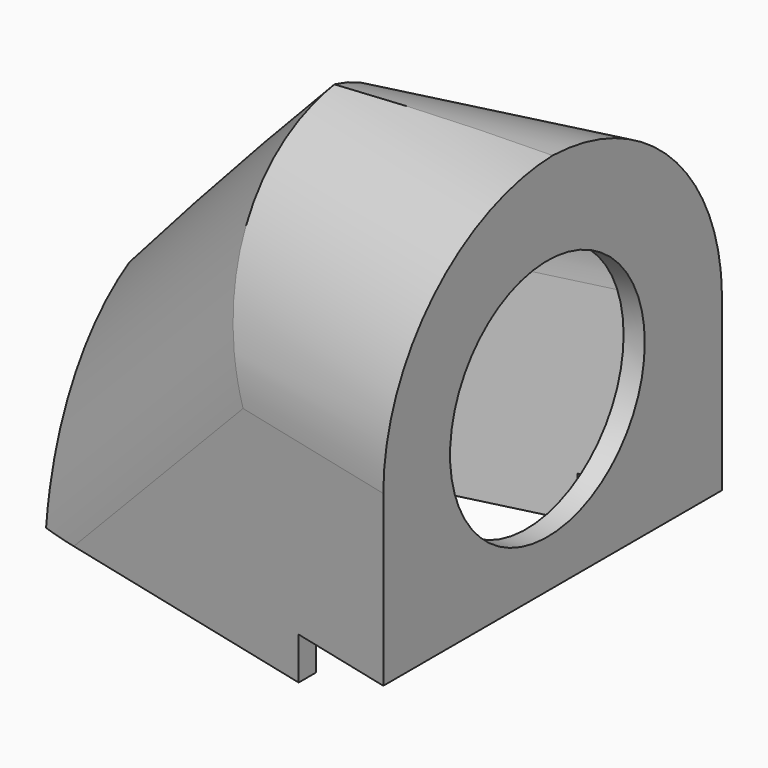
from build123d import *

# Parameters (mm, degrees)
F1_DEPTH    = 40
F2_SIZE     = 20
F3_T1_DEPTH = 120.6155281281
F3_T3_DEPTH = 120.6155281281
F3_T5_DEPTH = 112.8188914216
F3_T7_DEPTH = 112.8188914216
F5_T        = -2
F4_R        = 11.5
F6_DEPTH    = 5
F8_DEPTH    = 4


# Not quite as in the source:
# - a fillet or chamfer that OpenCascade refuses, or shapes differently, is made with other operations: its cross-section is extruded or revolved along the edge and cut away or added


with BuildPart() as f1:
    # F0 (on Top) → F1 (new body)
    with BuildSketch(Plane.XY):
        Polygon((-40, 10), (0, 0), (0, 40), (-40, 30), align=None)
    extrude(amount=F1_DEPTH)

    # F2
    f2_edges = [f1.edges().sort_by_distance(p)[0] for p in [
        (-40, 20, 40),
    ]]
    chamfer(f2_edges, length=F2_SIZE)

    # F3: fillet of radius 20 on 4 edges, made by hand

    # F3_s2 → F3_t1 (cut)
    with BuildSketch(Plane(origin=(57.9188897131, 14.4797224283, 0), x_dir=(0, 0, 1), z_dir=(-0.9701425001, -0.242535625, 0))):
        with BuildLine():
            ThreePointArc((40, 18.8057000058), (34.1421356237, 32.9478356295), (20, 38.8057000058))
            Line((20, 38.8057000058), (40, 38.8057000058))
            Line((40, 38.8057000058), (40, 18.8057000058))
        make_face()
    extrude(amount=F3_T1_DEPTH, mode=Mode.SUBTRACT)

    # F3_s4 → F3_t3 (cut)
    with BuildSketch(Plane(origin=(-68.5071250073, 17.1267812518, 0), x_dir=(0, 0, 1), z_dir=(0.9701425001, -0.242535625, 0))):
        with BuildLine():
            ThreePointArc((20, 0), (34.1421356237, -5.8578643763), (40, -20))
            Line((40, -20), (40, 0))
            Line((40, 0), (20, 0))
        make_face()
    extrude(amount=F3_T3_DEPTH, mode=Mode.SUBTRACT)

    # F3_s6 → F3_t5 (cut)
    with BuildSketch(Plane(origin=(-40.1875872415, 10.0468968104, -40.1875872415), x_dir=(0.242535625, 0.9701425001, 0), z_dir=(0.6963106238, -0.174077656, 0.6963106238))):
        with BuildLine():
            ThreePointArc((0, 26.2452181161), (4.6931480366, 39.1176803115), (16.5700282971, 45.948905439))
            Line((16.5700282971, 45.948905439), (0, 43.0644337539))
            Line((0, 43.0644337539), (0, 26.2452181161))
        make_face()
    extrude(amount=F3_T5_DEPTH, mode=Mode.SUBTRACT)

    # F3_s8 → F3_t7 (cut)
    with BuildSketch(Plane(origin=(-35.339102393, -8.8347755983, -35.339102393), x_dir=(-0.242535625, 0.9701425001, 0), z_dir=(0.6963106238, 0.174077656, 0.6963106238))):
        with BuildLine():
            ThreePointArc((22.2356717087, 39.1937001443), (34.1125519692, 32.3624750168), (38.8057000058, 19.4900128214))
            Line((38.8057000058, 19.4900128214), (38.8057000058, 36.3092284592))
            Line((38.8057000058, 36.3092284592), (22.2356717087, 39.1937001443))
        make_face()
    extrude(amount=F3_T7_DEPTH, mode=Mode.SUBTRACT)

    # F5
    f5_openings = [f1.faces().sort_by_distance(p)[0] for p in [
        (-17.771277, 20, 0),
    ]]
    offset(amount=F5_T, openings=f5_openings)

    # F4 (on face) → F6 (cut)
    with BuildSketch(Plane.YZ):
        with Locations((19.3844718719, 20)):
            Circle(F4_R)
    extrude(amount=-F6_DEPTH, mode=Mode.SUBTRACT)

    # F7 (on face) → F8 (cut)
    with BuildSketch(Plane.XY):
        Polygon((-10.0002693493, 2.5000673373), (0, 0), (0, 40), (-10.0040400222, 37.4989899944), align=None)
    extrude(amount=F8_DEPTH, mode=Mode.SUBTRACT)


solid = f1.part
